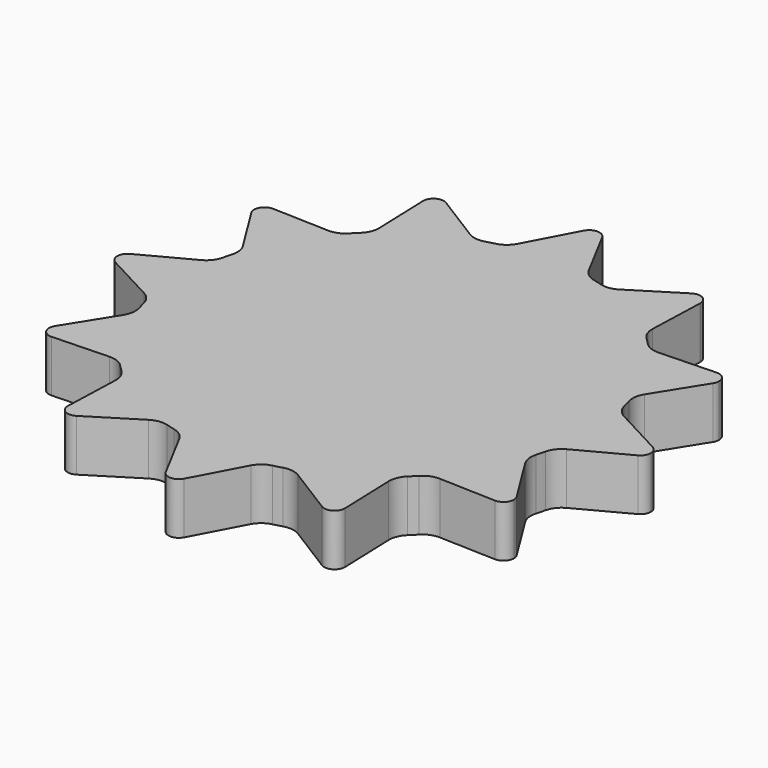
from build123d import *

# Parameters (mm, degrees)
F1_DEPTH = 6.35


with BuildPart() as f1:
    # F0 (on Top) → F1 (new body)
    with BuildSketch(Plane.XY):
        with BuildLine():
            ThreePointArc((-4.39292013, 25.9471153947), (-5.0763171932, 25.1352197323), (-6.031797544, 24.6734152153))
            ThreePointArc((-6.031797544, 24.6734152153), (-6.5740037456, 24.5345159877), (-7.1130177041, 24.3837031466))
            ThreePointArc((-7.1130177041, 24.3837031466), (-12.7, 21.9970452561), (-17.5603975113, 18.3519056026))
            ThreePointArc((-17.5603975113, 18.3519056026), (-17.9605122421, 17.9605122421), (-18.3519056026, 17.5603975113))
            ThreePointArc((-18.3519056026, 17.5603975113), (-21.9970452561, 12.7), (-24.3837031466, 7.1130177041))
            ThreePointArc((-24.3837031466, 7.1130177041), (-24.5345159877, 6.5740037456), (-24.6734152153, 6.031797544))
            ThreePointArc((-24.6734152153, 6.031797544), (-25.4, 0), (-24.6734152153, -6.031797544))
            ThreePointArc((-24.6734152153, -6.031797544), (-24.5345159877, -6.5740037456), (-24.3837031466, -7.1130177041))
            ThreePointArc((-24.3837031466, -7.1130177041), (-21.9970452561, -12.7), (-18.3519056026, -17.5603975113))
            ThreePointArc((-18.3519056026, -17.5603975113), (-17.9605122421, -17.9605122421), (-17.5603975113, -18.3519056026))
            ThreePointArc((-17.5603975113, -18.3519056026), (-12.7, -21.9970452561), (-7.1130177041, -24.3837031466))
            ThreePointArc((-7.1130177041, -24.3837031466), (-6.5740037456, -24.5345159877), (-6.031797544, -24.6734152153))
            ThreePointArc((-6.031797544, -24.6734152153), (0, -25.4), (6.031797544, -24.6734152153))
            ThreePointArc((6.031797544, -24.6734152153), (6.5740037456, -24.5345159877), (7.1130177041, -24.3837031466))
            ThreePointArc((7.1130177041, -24.3837031466), (12.7, -21.9970452561), (17.5603975113, -18.3519056026))
            ThreePointArc((17.5603975113, -18.3519056026), (17.9605122421, -17.9605122421), (18.3519056026, -17.5603975113))
            ThreePointArc((18.3519056026, -17.5603975113), (21.9970452561, -12.7), (24.3837031466, -7.1130177041))
            ThreePointArc((24.3837031466, -7.1130177041), (24.5345159877, -6.5740037456), (24.6734152153, -6.031797544))
            ThreePointArc((24.6734152153, -6.031797544), (25.4, 0), (24.6734152153, 6.031797544))
            ThreePointArc((24.6734152153, 6.031797544), (24.5345159877, 6.5740037456), (24.3837031466, 7.1130177041))
            ThreePointArc((24.3837031466, 7.1130177041), (21.9970452561, 12.7), (18.3519056026, 17.5603975113))
            ThreePointArc((18.3519056026, 17.5603975113), (17.9605122421, 17.9605122421), (17.5603975113, 18.3519056026))
            ThreePointArc((17.5603975113, 18.3519056026), (12.7, 21.9970452561), (7.1130177041, 24.3837031466))
            ThreePointArc((7.1130177041, 24.3837031466), (6.5740037456, 24.5345159877), (6.031797544, 24.6734152153))
            ThreePointArc((6.031797544, 24.6734152153), (5.0763171932, 25.1352197323), (4.39292013, 25.9471153947))
            Line((4.39292013, 25.9471153947), (1.1210285842, 32.0928206711))
            ThreePointArc((1.1210285842, 32.0928206711), (1.2321944453, 31.8035660076), (1.27, 31.496))
            ThreePointArc((1.27, 31.496), (0.8980256121, 30.5979743879), (0, 30.226))
            ThreePointArc((0, 30.226), (-1.0887750576, 30.8421889616), (-1.1210285842, 32.0928206711))
            Line((-1.1210285842, 32.0928206711), (-4.39292013, 25.9471153947))
        make_face()
        with BuildLine():
            ThreePointArc((-17.5603975113, 18.3519056026), (-12.7, 21.9970452561), (-7.1130177041, 24.3837031466))
            ThreePointArc((-7.1130177041, 24.3837031466), (-8.1713902192, 24.3058974145), (-9.169177268, 24.6673211518))
            Line((-9.169177268, 24.6673211518), (-15.0755711033, 28.3537122723))
            ThreePointArc((-15.0755711033, 28.3537122723), (-14.6373955027, 27.8923374573), (-14.478, 27.2763361176))
            ThreePointArc((-14.478, 27.2763361176), (-15.7261705603, 26.0065237395), (-17.0172495678, 27.2326836881))
            Line((-17.0172495678, 27.2326836881), (-16.7779381267, 20.2744010218))
            ThreePointArc((-16.7779381267, 20.2744010218), (-16.9638295132, 19.2295802213), (-17.5603975113, 18.3519056026))
        make_face()
        with BuildLine():
            ThreePointArc((1.1210285842, 32.0928206711), (0, 32.766), (-1.1210285842, 32.0928206711))
            ThreePointArc((-1.1210285842, 32.0928206711), (-1.0887750576, 30.8421889616), (0, 30.226))
            ThreePointArc((0, 30.226), (0.8980256121, 30.5979743879), (1.27, 31.496))
            ThreePointArc((1.27, 31.496), (1.2321944453, 31.8035660076), (1.1210285842, 32.0928206711))
        make_face()
        with BuildLine():
            ThreePointArc((-24.3837031466, 7.1130177041), (-21.9970452561, 12.7), (-18.3519056026, 17.5603975113))
            ThreePointArc((-18.3519056026, 17.5603975113), (-19.2295802213, 16.9638295132), (-20.2744010218, 16.7779381267))
            Line((-20.2744010218, 16.7779381267), (-27.2326836881, 17.0172495678))
            ThreePointArc((-27.2326836881, 17.0172495678), (-26.3630074294, 16.6304571986), (-26.0063361176, 15.748))
            ThreePointArc((-26.0063361176, 15.748), (-26.9265988709, 14.5271053042), (-28.3537122723, 15.0755711033))
            Line((-28.3537122723, 15.0755711033), (-24.6673211518, 9.169177268))
            ThreePointArc((-24.6673211518, 9.169177268), (-24.3058974145, 8.1713902192), (-24.3837031466, 7.1130177041))
        make_face()
        with BuildLine():
            ThreePointArc((-14.478, 27.2763361176), (-14.6373955027, 27.8923374573), (-15.0755711033, 28.3537122723))
            ThreePointArc((-15.0755711033, 28.3537122723), (-16.383, 28.3761883804), (-17.0172495678, 27.2326836881))
            ThreePointArc((-17.0172495678, 27.2326836881), (-15.7261705603, 26.0065237395), (-14.478, 27.2763361176))
        make_face()
        with BuildLine():
            ThreePointArc((-24.6734152153, -6.031797544), (-25.4, 0), (-24.6734152153, 6.031797544))
            ThreePointArc((-24.6734152153, 6.031797544), (-25.1352197323, 5.0763171932), (-25.9471153947, 4.39292013))
            Line((-25.9471153947, 4.39292013), (-32.0928206711, 1.1210285842))
            ThreePointArc((-32.0928206711, 1.1210285842), (-30.8421889616, 1.0887750576), (-30.226, 0))
            ThreePointArc((-30.226, 0), (-30.8421889616, -1.0887750576), (-32.0928206711, -1.1210285842))
            Line((-32.0928206711, -1.1210285842), (-25.9471153947, -4.39292013))
            ThreePointArc((-25.9471153947, -4.39292013), (-25.1352197323, -5.0763171932), (-24.6734152153, -6.031797544))
        make_face()
        with BuildLine():
            ThreePointArc((-26.0063361176, 15.748), (-26.3630074294, 16.6304571986), (-27.2326836881, 17.0172495678))
            ThreePointArc((-27.2326836881, 17.0172495678), (-28.3761883804, 16.383), (-28.3537122723, 15.0755711033))
            ThreePointArc((-28.3537122723, 15.0755711033), (-26.9265988709, 14.5271053042), (-26.0063361176, 15.748))
        make_face()
        with BuildLine():
            ThreePointArc((9.169177268, 24.6673211518), (8.1713902192, 24.3058974145), (7.1130177041, 24.3837031466))
            ThreePointArc((7.1130177041, 24.3837031466), (12.7, 21.9970452561), (17.5603975113, 18.3519056026))
            ThreePointArc((17.5603975113, 18.3519056026), (16.9638295132, 19.2295802213), (16.7779381267, 20.2744010218))
            Line((16.7779381267, 20.2744010218), (17.0172495678, 27.2326836881))
            ThreePointArc((17.0172495678, 27.2326836881), (15.113, 26.1764838548), (15.0755711033, 28.3537122723))
            Line((15.0755711033, 28.3537122723), (9.169177268, 24.6673211518))
        make_face()
        with BuildLine():
            ThreePointArc((-18.3519056026, -17.5603975113), (-21.9970452561, -12.7), (-24.3837031466, -7.1130177041))
            ThreePointArc((-24.3837031466, -7.1130177041), (-24.3058974145, -8.1713902192), (-24.6673211518, -9.169177268))
            Line((-24.6673211518, -9.169177268), (-28.3537122723, -15.0755711033))
            ThreePointArc((-28.3537122723, -15.0755711033), (-26.9265988709, -14.5271053042), (-26.0063361176, -15.748))
            ThreePointArc((-26.0063361176, -15.748), (-26.3630074294, -16.6304571986), (-27.2326836881, -17.0172495678))
            Line((-27.2326836881, -17.0172495678), (-20.2744010218, -16.7779381267))
            ThreePointArc((-20.2744010218, -16.7779381267), (-19.2295802213, -16.9638295132), (-18.3519056026, -17.5603975113))
        make_face()
        with BuildLine():
            ThreePointArc((-30.226, 0), (-30.8421889616, 1.0887750576), (-32.0928206711, 1.1210285842))
            ThreePointArc((-32.0928206711, 1.1210285842), (-32.766, 0), (-32.0928206711, -1.1210285842))
            ThreePointArc((-32.0928206711, -1.1210285842), (-30.8421889616, -1.0887750576), (-30.226, 0))
        make_face()
        with BuildLine():
            ThreePointArc((20.2744010218, 16.7779381267), (19.2295802213, 16.9638295132), (18.3519056026, 17.5603975113))
            ThreePointArc((18.3519056026, 17.5603975113), (21.9970452561, 12.7), (24.3837031466, 7.1130177041))
            ThreePointArc((24.3837031466, 7.1130177041), (24.3058974145, 8.1713902192), (24.6673211518, 9.169177268))
            Line((24.6673211518, 9.169177268), (28.3537122723, 15.0755711033))
            ThreePointArc((28.3537122723, 15.0755711033), (26.1764838548, 15.113), (27.2326836881, 17.0172495678))
            Line((27.2326836881, 17.0172495678), (20.2744010218, 16.7779381267))
        make_face()
        with BuildLine():
            ThreePointArc((17.018, 27.2763361176), (16.3640013397, 28.3869406149), (15.0755711033, 28.3537122723))
            ThreePointArc((15.0755711033, 28.3537122723), (15.113, 26.1764838548), (17.0172495678, 27.2326836881))
            ThreePointArc((17.0172495678, 27.2326836881), (17.0178123781, 27.2545066779), (17.018, 27.2763361176))
        make_face()
        with BuildLine():
            ThreePointArc((-7.1130177041, -24.3837031466), (-12.7, -21.9970452561), (-17.5603975113, -18.3519056026))
            ThreePointArc((-17.5603975113, -18.3519056026), (-16.9638295132, -19.2295802213), (-16.7779381267, -20.2744010218))
            Line((-16.7779381267, -20.2744010218), (-17.0172495678, -27.2326836881))
            ThreePointArc((-17.0172495678, -27.2326836881), (-15.7261705603, -26.0065237395), (-14.478, -27.2763361176))
            ThreePointArc((-14.478, -27.2763361176), (-14.6373955027, -27.8923374573), (-15.0755711033, -28.3537122723))
            Line((-15.0755711033, -28.3537122723), (-9.169177268, -24.6673211518))
            ThreePointArc((-9.169177268, -24.6673211518), (-8.1713902192, -24.3058974145), (-7.1130177041, -24.3837031466))
        make_face()
        with BuildLine():
            ThreePointArc((-26.0063361176, -15.748), (-26.9265988709, -14.5271053042), (-28.3537122723, -15.0755711033))
            ThreePointArc((-28.3537122723, -15.0755711033), (-28.3761883804, -16.383), (-27.2326836881, -17.0172495678))
            ThreePointArc((-27.2326836881, -17.0172495678), (-26.3630074294, -16.6304571986), (-26.0063361176, -15.748))
        make_face()
        with BuildLine():
            ThreePointArc((25.9471153947, 4.39292013), (25.1352197323, 5.0763171932), (24.6734152153, 6.031797544))
            ThreePointArc((24.6734152153, 6.031797544), (25.4, 0), (24.6734152153, -6.031797544))
            ThreePointArc((24.6734152153, -6.031797544), (25.1352197323, -5.0763171932), (25.9471153947, -4.39292013))
            Line((25.9471153947, -4.39292013), (32.0928206711, -1.1210285842))
            ThreePointArc((32.0928206711, -1.1210285842), (30.226, 0), (32.0928206711, 1.1210285842))
            Line((32.0928206711, 1.1210285842), (25.9471153947, 4.39292013))
        make_face()
        with BuildLine():
            ThreePointArc((28.5463361176, 15.748), (28.1587933162, 16.6613286882), (27.2326836881, 17.0172495678))
            ThreePointArc((27.2326836881, 17.0172495678), (26.1764838548, 15.113), (28.3537122723, 15.0755711033))
            ThreePointArc((28.3537122723, 15.0755711033), (28.4972308134, 15.3982627533), (28.5463361176, 15.748))
        make_face()
        with BuildLine():
            ThreePointArc((6.031797544, -24.6734152153), (0, -25.4), (-6.031797544, -24.6734152153))
            ThreePointArc((-6.031797544, -24.6734152153), (-5.0763171932, -25.1352197323), (-4.39292013, -25.9471153947))
            Line((-4.39292013, -25.9471153947), (-1.1210285842, -32.0928206711))
            ThreePointArc((-1.1210285842, -32.0928206711), (-0.3075660076, -30.2638055547), (1.27, -31.496))
            ThreePointArc((1.27, -31.496), (1.2321944453, -31.8035660076), (1.1210285842, -32.0928206711))
            Line((1.1210285842, -32.0928206711), (4.39292013, -25.9471153947))
            ThreePointArc((4.39292013, -25.9471153947), (5.0763171932, -25.1352197323), (6.031797544, -24.6734152153))
        make_face()
        with BuildLine():
            ThreePointArc((-14.478, -27.2763361176), (-15.7261705603, -26.0065237395), (-17.0172495678, -27.2326836881))
            ThreePointArc((-17.0172495678, -27.2326836881), (-16.383, -28.3761883804), (-15.0755711033, -28.3537122723))
            ThreePointArc((-15.0755711033, -28.3537122723), (-14.6373955027, -27.8923374573), (-14.478, -27.2763361176))
        make_face()
        with BuildLine():
            ThreePointArc((24.6673211518, -9.169177268), (24.3058974145, -8.1713902192), (24.3837031466, -7.1130177041))
            ThreePointArc((24.3837031466, -7.1130177041), (21.9970452561, -12.7), (18.3519056026, -17.5603975113))
            ThreePointArc((18.3519056026, -17.5603975113), (19.2295802213, -16.9638295132), (20.2744010218, -16.7779381267))
            Line((20.2744010218, -16.7779381267), (27.2326836881, -17.0172495678))
            ThreePointArc((27.2326836881, -17.0172495678), (26.1764838548, -15.113), (28.3537122723, -15.0755711033))
            Line((28.3537122723, -15.0755711033), (24.6673211518, -9.169177268))
        make_face()
        with BuildLine():
            ThreePointArc((32.766, 0), (32.5847750576, 0.6538110384), (32.0928206711, 1.1210285842))
            ThreePointArc((32.0928206711, 1.1210285842), (30.226, 0), (32.0928206711, -1.1210285842))
            ThreePointArc((32.0928206711, -1.1210285842), (32.5847750576, -0.6538110384), (32.766, 0))
        make_face()
        with BuildLine():
            ThreePointArc((17.5603975113, -18.3519056026), (12.7, -21.9970452561), (7.1130177041, -24.3837031466))
            ThreePointArc((7.1130177041, -24.3837031466), (8.1713902192, -24.3058974145), (9.169177268, -24.6673211518))
            Line((9.169177268, -24.6673211518), (15.0755711033, -28.3537122723))
            ThreePointArc((15.0755711033, -28.3537122723), (15.113, -26.1764838548), (17.0172495678, -27.2326836881))
            Line((17.0172495678, -27.2326836881), (16.7779381267, -20.2744010218))
            ThreePointArc((16.7779381267, -20.2744010218), (16.9638295132, -19.2295802213), (17.5603975113, -18.3519056026))
        make_face()
        with BuildLine():
            ThreePointArc((1.27, -31.496), (-0.3075660076, -30.2638055547), (-1.1210285842, -32.0928206711))
            ThreePointArc((-1.1210285842, -32.0928206711), (0, -32.766), (1.1210285842, -32.0928206711))
            ThreePointArc((1.1210285842, -32.0928206711), (1.2321944453, -31.8035660076), (1.27, -31.496))
        make_face()
        with BuildLine():
            ThreePointArc((28.5463361176, -15.748), (28.4972308134, -15.3982627533), (28.3537122723, -15.0755711033))
            ThreePointArc((28.3537122723, -15.0755711033), (26.1764838548, -15.113), (27.2326836881, -17.0172495678))
            ThreePointArc((27.2326836881, -17.0172495678), (28.1587933162, -16.6613286882), (28.5463361176, -15.748))
        make_face()
        with BuildLine():
            ThreePointArc((17.0172495678, -27.2326836881), (15.113, -26.1764838548), (15.0755711033, -28.3537122723))
            ThreePointArc((15.0755711033, -28.3537122723), (16.3640013397, -28.3869406149), (17.018, -27.2763361176))
            ThreePointArc((17.018, -27.2763361176), (17.0178123781, -27.2545066779), (17.0172495678, -27.2326836881))
        make_face()
    extrude(amount=F1_DEPTH)


solid = f1.part
